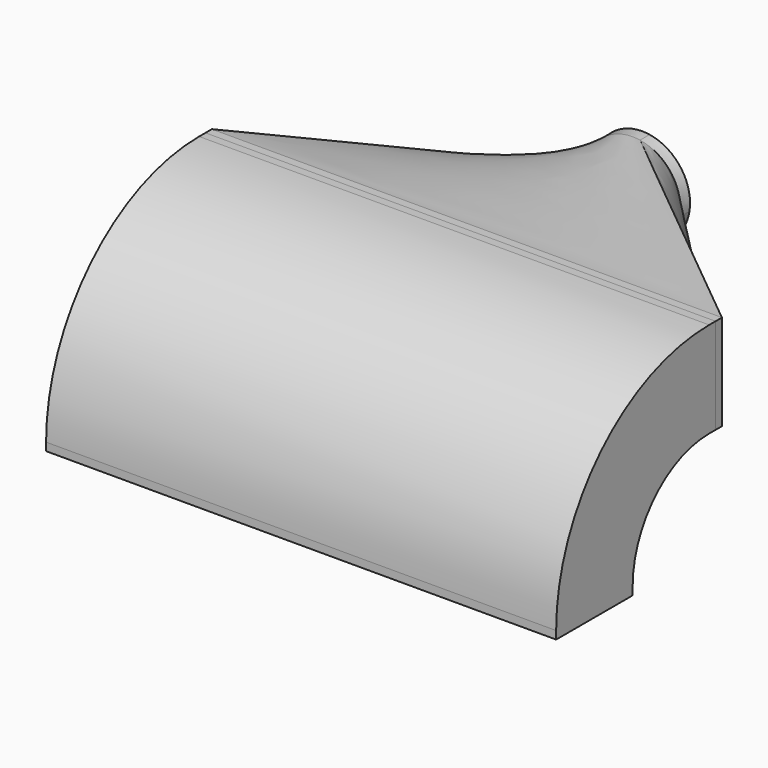
from build123d import *

# Parameters (mm, degrees)
F0_W      = 2438.4
F0_H      = 457.2
F1_DEPTH  = 38.1
F2_W      = 2438.4
F2_H      = 457.2
F3_ANGLE  = 90
F4_DEPTH  = 38.1
F5_W      = 2438.4
F5_H      = 457.2
F6_DEPTH  = 38.1
F6_FACE_W = 2438.4
F6_FACE_H = 457.2
F10_DEPTH = 57.15


# Not quite as in the source:
# - the arcs of a loft's sections are written as splines that run evenly, so that the points pair up as in the source's solid


with BuildPart() as f1:
    # F0 (on Top) → F1 (new body)
    with BuildSketch(Plane.XY):
        Rectangle(F0_W, F0_H)
    extrude(amount=F1_DEPTH)

    # F2 (on face) → F3 (revolve)
    with BuildSketch(Plane.XY.offset(38.1)):
        Rectangle(F2_W, F2_H)
    revolve(axis=Axis((-103.2055318356, 685.8, 38.1), (-1, 0, 0)), revolution_arc=F3_ANGLE)

    # F4 (add): a face of the model
    f4_faces = [f1.faces().sort_by_distance(p)[0] for p in [
        (0, 685.8, 723.9),
    ]]
    extrude(f4_faces, amount=F4_DEPTH)


with BuildPart() as f6:
    # F5 (on face) → F6 (new body)
    with BuildSketch(Plane(origin=(0, 723.9, 0), x_dir=(-1, 0, 0), z_dir=(0, 1, 0))):
        with Locations((0, 723.9)):
            Rectangle(F5_W, F5_H)
    extrude(amount=F6_DEPTH)

    # F6_face (on face) → F9 section 0
    with BuildSketch(Plane(origin=(0, 762, 723.9), x_dir=(-1, 0, 0), z_dir=(0, 1, 0))):
        Rectangle(F6_FACE_W, F6_FACE_H)
    # F8 (on offset) → F9 section 1
    with BuildSketch(Plane(origin=(0, 1752.6, 0), x_dir=(-1, 0, 0), z_dir=(0, 1, 0))):
        with BuildLine():
            add(Edge.make_bspline(
                [(-225.8595509155, 650.5094451695), (-223.5497895031, 635.7269721299), (-219.7841746904, 621.1723506338), (-209.4855798503, 593.076710899), (-202.952854476, 579.5363873802), (-187.3709568448, 553.9897536684), (-178.3221698812, 541.9840751662), (-158.0557730466, 519.9681902843), (-146.8386643022, 509.9585282907), (-122.6665945289, 492.3194503481), (-109.7122312021, 484.69047056), (-82.5634075757, 472.1060594298), (-68.3696185843, 467.1509392621), (-39.2873551715, 460.1048068067), (-24.3995998664, 458.0139687485), (5.4984882594, 456.7768938866), (20.508081791, 457.6306876721), (35.2905548305, 459.9404490845)],
                knots=[0, 0, 0, 0, 0.125, 0.125, 0.25, 0.25, 0.375, 0.375, 0.5, 0.5, 0.625, 0.625, 0.75, 0.75, 0.875, 0.875, 1, 1, 1, 1], degree=3))
            add(Edge.make_bspline(
                [(35.2905548305, 459.9404490845), (50.0730278701, 462.2502104969), (64.6276493662, 466.0158253096), (92.723289101, 476.3144201497), (106.2636126198, 482.847145524), (131.8102463316, 498.4290431552), (143.8159248338, 507.4778301188), (165.8318097157, 527.7442269534), (175.8414717093, 538.9613356978), (193.4805496519, 563.1334054711), (201.10952944, 576.0877687979), (213.6939405702, 603.2365924243), (218.6490607379, 617.4303814157), (225.6951931933, 646.5126448285), (227.7860312515, 661.4004001336), (229.0231061134, 691.2984882594), (228.1693123279, 706.308081791), (225.8595509155, 721.0905548305)],
                knots=[0, 0, 0, 0, 0.125, 0.125, 0.25, 0.25, 0.375, 0.375, 0.5, 0.5, 0.625, 0.625, 0.75, 0.75, 0.875, 0.875, 1, 1, 1, 1], degree=3))
            add(Edge.make_bspline(
                [(225.8595509155, 721.0905548305), (223.5497895031, 735.8730278701), (219.7841746904, 750.4276493662), (209.4855798503, 778.523289101), (202.952854476, 792.0636126198), (187.3709568448, 817.6102463316), (178.3221698812, 829.6159248338), (158.0557730466, 851.6318097157), (146.8386643022, 861.6414717093), (122.6665945289, 879.2805496519), (109.7122312021, 886.90952944), (82.5634075757, 899.4939405702), (68.3696185843, 904.4490607379), (39.2873551715, 911.4951931933), (24.3995998664, 913.5860312515), (-5.4984882594, 914.8231061134), (-20.508081791, 913.9693123279), (-35.2905548305, 911.6595509155)],
                knots=[0, 0, 0, 0, 0.125, 0.125, 0.25, 0.25, 0.375, 0.375, 0.5, 0.5, 0.625, 0.625, 0.75, 0.75, 0.875, 0.875, 1, 1, 1, 1], degree=3))
            add(Edge.make_bspline(
                [(-35.2905548305, 911.6595509155), (-50.0730278701, 909.3497895031), (-64.6276493662, 905.5841746904), (-92.723289101, 895.2855798503), (-106.2636126198, 888.752854476), (-131.8102463316, 873.1709568448), (-143.8159248338, 864.1221698812), (-165.8318097157, 843.8557730466), (-175.8414717093, 832.6386643022), (-193.4805496519, 808.4665945289), (-201.10952944, 795.5122312021), (-213.6939405702, 768.3634075757), (-218.6490607379, 754.1696185843), (-225.6951931933, 725.0873551715), (-227.7860312515, 710.1995998664), (-229.0231061134, 680.3015117406), (-228.1693123279, 665.291918209), (-225.8595509155, 650.5094451695)],
                knots=[0, 0, 0, 0, 0.125, 0.125, 0.25, 0.25, 0.375, 0.375, 0.5, 0.5, 0.625, 0.625, 0.75, 0.75, 0.875, 0.875, 1, 1, 1, 1], degree=3))
        make_face()
    loft(ruled=True)

    # F10 (add): a face of the model
    f10_faces = [f6.faces().sort_by_distance(p)[0] for p in [
        (0, 1752.6, 685.8),
    ]]
    extrude(f10_faces, amount=F10_DEPTH)


solid = Compound([f1.part, f6.part])
